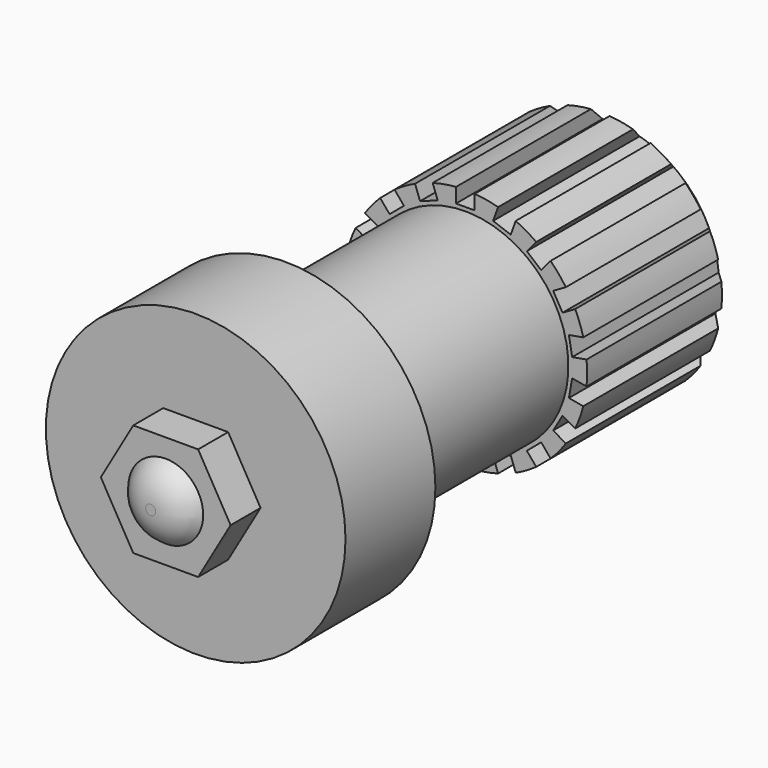
from build123d import *

# Parameters (mm, degrees)
F0_R             = 8
F1_DEPTH         = 6
F3_DEPTH         = 2
F4_R             = 2
F5_DEPTH         = 1
F7_R             = 5.5
F8_DEPTH         = 22
F9_R             = 6.5
F9_R_2           = 5.5
F10_DEPTH        = 10
F11_SIZE         = 1
F12_W            = 1
F12_H            = 2
F13_DEPTH        = 20
F13_COPIES_COUNT = 18


# Not quite as in the source:
# - a fillet or chamfer that OpenCascade refuses, or shapes differently, is made with other operations: its cross-section is extruded or revolved along the edge and cut away or added
# - a pattern or mirror of a feature is missing from the dataset's text; its kind, count and spacing are read off the source's solid


with BuildPart() as f1:
    # F0 (on Front) → F1 (new body)
    with BuildSketch(Plane.XZ):
        Circle(F0_R)
    extrude(amount=-F1_DEPTH)

    # F2 (on face) → F3 (join)
    with BuildSketch(Plane.XZ):
        Polygon((-1.7320508076, 3), (-3.4641016151, 0), (-1.7320508076, -3), (1.7320508076, -3), (3.4641016151, 0), (1.7320508076, 3), align=None)
    extrude(amount=F3_DEPTH)

    # F4 (on face) → F5 (join)
    with BuildSketch(Plane.XZ.offset(2)):
        Circle(F4_R)
    extrude(amount=F5_DEPTH)

    # F6: fillet of radius 2 on 1 edges, made by hand

    # F6_s1 → F6_t2 (revolve, cut)
    with BuildSketch(Plane.XY):
        with BuildLine():
            ThreePointArc((2, -2), (1.2679491924, -2.7320508076), (0.2679491924, -3))
            Line((0.2679491924, -3), (2, -3))
            Line((2, -3), (2, -2))
        make_face()
    revolve(axis=Axis((0, -3, 0), (0, -1, 0)), mode=Mode.SUBTRACT)

    # F7 (on face) → F8 (join)
    with BuildSketch(Plane(origin=(0, 6, 0), x_dir=(-1, 0, 0), z_dir=(0, 1, 0))):
        Circle(F7_R)
    extrude(amount=F8_DEPTH)

    # F9 (on face) → F10 (join)
    with BuildSketch(Plane(origin=(0, 28, 0), x_dir=(-1, 0, 0), z_dir=(0, 1, 0))):
        Circle(F9_R)
        Circle(F9_R_2, mode=Mode.SUBTRACT)
    extrude(amount=-F10_DEPTH)

    # F11
    f11_edges = [f1.edges().sort_by_distance(p)[0] for p in [
        (6.5, 28, 0),
    ]]
    chamfer(f11_edges, length=F11_SIZE)

    # F12 (on face) → F13 (cut)
    with BuildSketch(Plane(origin=(0, 28, 0), x_dir=(-1, 0, 0), z_dir=(0, 1, 0))):
        with Locations((0, 6.7)):
            Rectangle(F12_W, F12_H)
    f13 = extrude(amount=-F13_DEPTH, mode=Mode.SUBTRACT)

    # F13_copies: F13 ×18 about axis
    f13_copies_axis = Axis((0, 0, 0), (0, 1, 0))
    for i in range(1, F13_COPIES_COUNT):
        add(f13.rotate(f13_copies_axis, i * 360 / F13_COPIES_COUNT), mode=Mode.SUBTRACT)


solid = f1.part
